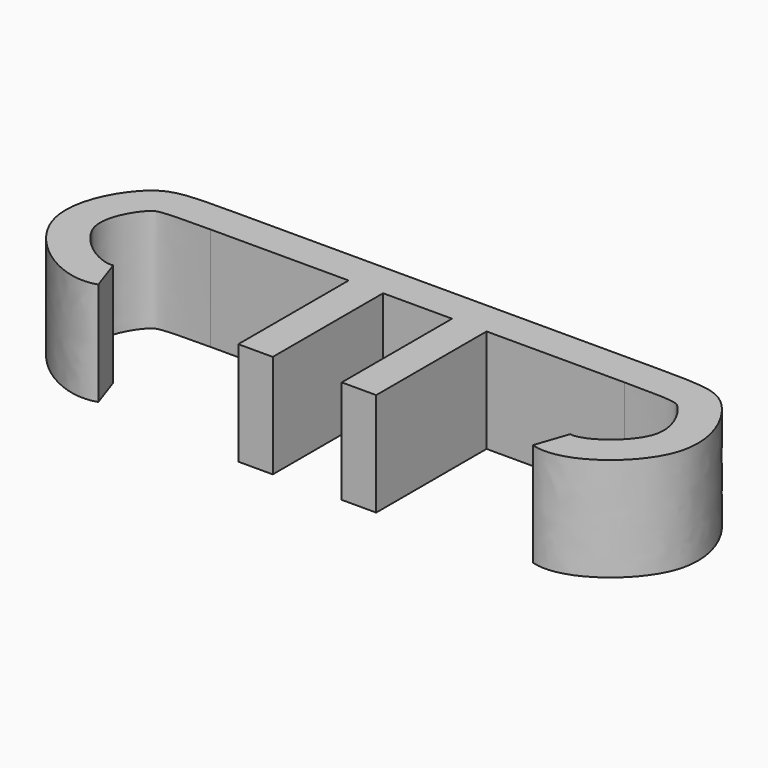
from build123d import *

# Parameters (mm, degrees)
F0_W     = 1
F0_H     = 1
F1_DEPTH = 3


# Not quite as in the source:
# - ends of sketch curves that miss each other by under 0.0002 mm in the source are joined
# - the dataset's text gives a spline's control points without its knots; the knots are read off the source's solid


with BuildPart() as f1:
    # F0 (on Top) → F1 (new body)
    with BuildSketch(Plane.XY):
        with Locations((0.5, -0.5)):
            Rectangle(F0_W, F0_H)
        with Locations((-0.5, -0.5)):
            Rectangle(F0_W, F0_H)
        Polygon((2, 0), (1, 0), (1, -1), (1, -5), (2, -5), (2, -1), align=None)
        Polygon((-1, -1), (-1, 0), (-2, 0), (-2, -1), (-2, -5), (-1, -5), align=None)
        with BuildLine():
            Line((6, 0), (2, 0))
            Line((2, 0), (2, -1))
            Line((2, -1), (6, -1))
            add(Edge.make_bspline(
                [(6, -1), (6.2943328716, -1), (6.7928790283, -1.0001284078), (7.2918933464, -1.0221779319), (7.4969615527, -1.0616895732), (7.56024585, -1.085258147), (7.5844634078, -1.0978186915), (7.6150443946, -1.1182344461), (7.6731849802, -1.1697526134), (7.7575411055, -1.2621427239), (7.8755473485, -1.4166571253), (8.0187330203, -1.659050071), (8.1368085957, -1.9798232644), (8.1720854573, -2.2348468695), (8.1618492839, -2.4205343228), (8.1357439574, -2.551784525), (8.0876272471, -2.6853118112), (8.0024166775, -2.8475491469), (7.8841123581, -3.0179740605), (7.6881815621, -3.2443388545), (7.3889123533, -3.5000214004), (7.0125685263, -3.7045676762), (6.7646613516, -3.7611825156), (6.6590556256, -3.7581499322), (6.6348866575, -3.7523734664), (6.6273172151, -3.7500032276)],
                knots=[0, 0, 0, 0, 0.0625, 0.125, 0.1875, 0.21875, 0.25, 0.28125, 0.3125, 0.34375, 0.375, 0.4375, 0.5, 0.5625, 0.59375, 0.625, 0.65625, 0.6875, 0.71875, 0.75, 0.8125, 0.875, 0.9375, 0.96875, 0.9966456355, 0.9966456355, 0.9966456355, 0.9966456355], degree=3))
            Line((6.6273172151, -3.7500032276), (6.3035145558, -4.6961655705))
            add(Edge.make_bspline(
                [(6, 0), (7.4849501429, 0), (8.3781624755, -0.0030244964), (9.961931742, -3.0861209791), (7.2766393676, -5.0262618498), (6.3035145558, -4.6961655705)],
                knots=[0, 0, 0, 0, 0.3151779178, 0.6343970778, 1, 1, 1, 1], degree=3))
        make_face()
        with BuildLine():
            Line((-2, -1), (-2, 0))
            Line((-2, 0), (-6, 0))
            add(Edge.make_bspline(
                [(-6, 0), (-7.4849501429, 0), (-8.3781624755, -0.0030244964), (-9.961931742, -3.0861209791), (-7.2766393676, -5.0262618498), (-6.3035145558, -4.6961655705)],
                knots=[0, 0, 0, 0, 0.3151779178, 0.6343970778, 1, 1, 1, 1], degree=3))
            Line((-6.3035145558, -4.6961655705), (-6.6273182258, -3.75))
            add(Edge.make_bspline(
                [(-6, -1), (-6.2943328716, -1), (-6.7928790283, -1.0001284078), (-7.2918933464, -1.0221779319), (-7.4969615527, -1.0616895732), (-7.56024585, -1.085258147), (-7.5844634078, -1.0978186915), (-7.6150443946, -1.1182344461), (-7.6731849802, -1.1697526134), (-7.7575411055, -1.2621427239), (-7.8755473485, -1.4166571253), (-8.0187330203, -1.659050071), (-8.1368085957, -1.9798232644), (-8.1720854573, -2.2348468695), (-8.1618492839, -2.4205343228), (-8.1357439574, -2.551784525), (-8.0876272471, -2.6853118112), (-8.0024166775, -2.8475491469), (-7.8841123581, -3.0179740605), (-7.6881815621, -3.2443388545), (-7.3889123533, -3.5000214004), (-7.0125685263, -3.7045676762), (-6.7646613516, -3.7611825156), (-6.6590556256, -3.7581499322), (-6.6348866575, -3.7523734664), (-6.6273182258, -3.75)],
                knots=[0, 0, 0, 0, 0.0625, 0.125, 0.1875, 0.21875, 0.25, 0.28125, 0.3125, 0.34375, 0.375, 0.4375, 0.5, 0.5625, 0.59375, 0.625, 0.65625, 0.6875, 0.71875, 0.75, 0.8125, 0.875, 0.9375, 0.96875, 0.9966456355, 0.9966456355, 0.9966456355, 0.9966456355], degree=3))
            Line((-6, -1), (-2, -1))
        make_face()
    extrude(amount=F1_DEPTH)


solid = f1.part
